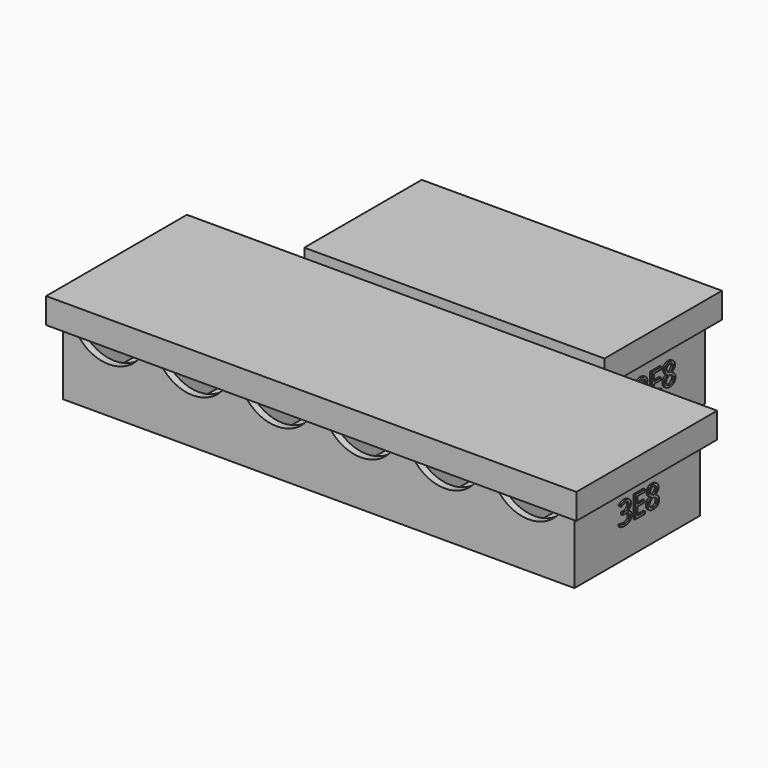
from build123d import *

# Parameters (mm, degrees)
F0_W          = 140
F0_H          = 43
F1_DEPTH      = 2
F0_W_2        = 77
F0_H_2        = 35
F2_W          = 140
F2_H          = 43
F2_W_2        = 21
F2_H_2        = 39
F3_DEPTH      = 21
F5_DEPTH      = 84.001
F7_W          = 145.2
F7_H          = 48.2
F8_DEPTH      = 2
F9_W          = 145.2
F9_H          = 48.2
F9_W_2        = 141.2
F9_H_2        = 44.2
F10_DEPTH     = 5
F11_W         = 77
F11_H         = 35
F11_W_2       = 23
F11_H_2       = 31
F12_DEPTH     = 23
F14_DEPTH     = 35.001
F16_W         = 82.2
F16_H         = 40.2
F17_DEPTH     = 2
F18_W         = 82.2
F18_H         = 40.2
F18_W_2       = 78.2
F18_H_2       = 36.2
F19_DEPTH     = 5
F20_TEXT_SIZE = 8.3333333333
F21_DEPTH     = 0.5
F22_TEXT_SIZE = 8.3333333333
F23_DEPTH     = 0.5


# Not quite as in the source:
# - Text() gives the source's letters only with a copy of the font that has no kerning and outlines rounded to 1/6400 em; it was checked with that copy


with BuildPart() as f1:
    # F0 (on Top) → F1 (new body)
    with BuildSketch(Plane.XY):
        Rectangle(F0_W, F0_H)
    extrude(amount=F1_DEPTH)

    # F2 (on face) → F3 (join)
    with BuildSketch(Plane.XY.offset(2)):
        Rectangle(F2_W, F2_H)
        with Locations((-57.5, 0)):
            Rectangle(F2_W_2, F2_H_2, mode=Mode.SUBTRACT)
        with Locations((-34.5, 0)):
            Rectangle(F2_W_2, F2_H_2, mode=Mode.SUBTRACT)
        with Locations((-11.5, 0)):
            Rectangle(F2_W_2, F2_H_2, mode=Mode.SUBTRACT)
        with Locations((11.5, 0)):
            Rectangle(F2_W_2, F2_H_2, mode=Mode.SUBTRACT)
        with Locations((34.5, 0)):
            Rectangle(F2_W_2, F2_H_2, mode=Mode.SUBTRACT)
        with Locations((57.5, 0)):
            Rectangle(F2_W_2, F2_H_2, mode=Mode.SUBTRACT)
    extrude(amount=F3_DEPTH)

    # F4 (on face) → F5 (cut, through all)
    with BuildSketch(Plane.XZ.offset(21.5)):
        with BuildLine():
            Line((-47, 23), (-68, 23))
            ThreePointArc((-68, 23), (-57.5, 12.5), (-47, 23))
        make_face()
        with BuildLine():
            Line((-24, 23), (-45, 23))
            ThreePointArc((-45, 23), (-34.5, 12.5), (-24, 23))
        make_face()
        with BuildLine():
            Line((-1, 23), (-22, 23))
            ThreePointArc((-22, 23), (-11.5, 12.5), (-1, 23))
        make_face()
        with BuildLine():
            Line((22, 23), (1, 23))
            ThreePointArc((1, 23), (11.5, 12.5), (22, 23))
        make_face()
        with BuildLine():
            Line((45, 23), (24, 23))
            ThreePointArc((24, 23), (34.5, 12.5), (45, 23))
        make_face()
        with BuildLine():
            Line((68, 23), (47, 23))
            ThreePointArc((47, 23), (57.5, 12.5), (68, 23))
        make_face()
    extrude(amount=-F5_DEPTH, mode=Mode.SUBTRACT)

    # F20 (on face) → F21 (join)
    with BuildSketch(Plane.YZ.offset(70)):
        with Locations((-6.8658854167, 8.5)):
            Text('3E8', F20_TEXT_SIZE, font='Open Sans', text_align=(TextAlign.LEFT, TextAlign.BOTTOM))
    extrude(amount=F21_DEPTH)


with BuildPart() as f1b:
    # F0 (on Top) → F1, piece 2 (new body)
    with BuildSketch(Plane.XY):
        with Locations((0, 45)):
            Rectangle(F0_W_2, F0_H_2)
    extrude(amount=F1_DEPTH)

    # F11 (on face) → F12 (join)
    with BuildSketch(Plane.XY.offset(2)):
        with Locations((0, 45)):
            Rectangle(F11_W, F11_H)
        with Locations((-25, 45)):
            Rectangle(F11_W_2, F11_H_2, mode=Mode.SUBTRACT)
        with Locations((0, 45)):
            Rectangle(F11_W_2, F11_H_2, mode=Mode.SUBTRACT)
        with Locations((25, 45)):
            Rectangle(F11_W_2, F11_H_2, mode=Mode.SUBTRACT)
    extrude(amount=F12_DEPTH)

    # F13 (on face) → F14 (cut, through all)
    with BuildSketch(Plane.XZ.offset(-27.5)):
        with BuildLine():
            Line((-13.5, 25), (-36.5, 25))
            ThreePointArc((-36.5, 25), (-25, 13.5), (-13.5, 25))
        make_face()
        with BuildLine():
            Line((11.5, 25), (-11.5, 25))
            ThreePointArc((-11.5, 25), (0, 13.5), (11.5, 25))
        make_face()
        with BuildLine():
            Line((36.5, 25), (13.5, 25))
            ThreePointArc((13.5, 25), (25, 13.5), (36.5, 25))
        make_face()
    extrude(amount=-F14_DEPTH, mode=Mode.SUBTRACT)

    # F22 (on face) → F23 (join)
    with BuildSketch(Plane.YZ.offset(38.5)):
        with Locations((38.1341145833, 9.5)):
            Text('3E8', F22_TEXT_SIZE, font='Open Sans', text_align=(TextAlign.LEFT, TextAlign.BOTTOM))
    extrude(amount=F23_DEPTH)


with BuildPart() as f8:
    # F7 (on offset) → F8 (new body)
    with BuildSketch(Plane.XY.offset(23.1)):
        Rectangle(F7_W, F7_H)
    extrude(amount=F8_DEPTH)

    # F9 (on face) → F10 (join)
    with BuildSketch(Plane(origin=(0, 0, 23.1), x_dir=(1, 0, 0), z_dir=(0, 0, -1))):
        Rectangle(F9_W, F9_H)
        Rectangle(F9_W_2, F9_H_2, mode=Mode.SUBTRACT)
    extrude(amount=F10_DEPTH)


with BuildPart() as f17:
    # F16 (on offset) → F17 (new body)
    with BuildSketch(Plane.XY.offset(25.1)):
        with Locations((0, 45)):
            Rectangle(F16_W, F16_H)
    extrude(amount=F17_DEPTH)

    # F18 (on face) → F19 (join)
    with BuildSketch(Plane(origin=(0, 0, 25.1), x_dir=(1, 0, 0), z_dir=(0, 0, -1))):
        with Locations((0, -45)):
            Rectangle(F18_W, F18_H)
        with Locations((0, -45)):
            Rectangle(F18_W_2, F18_H_2, mode=Mode.SUBTRACT)
    extrude(amount=F19_DEPTH)


solid = Compound([f1.part, f1b.part, f8.part, f17.part])
